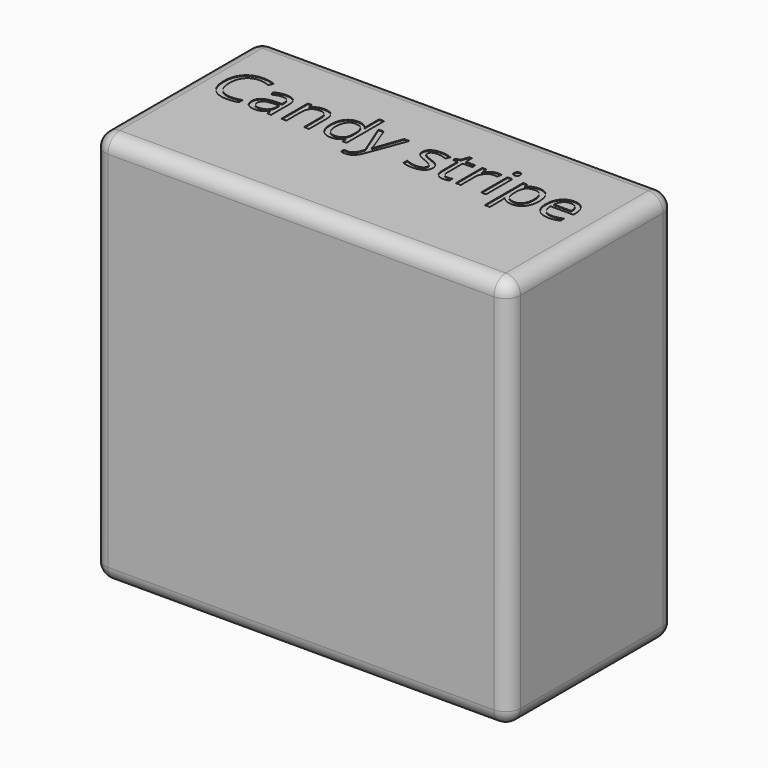
from build123d import *

# Parameters (mm, degrees)
F0_W         = 560
F0_H         = 280
F1_DEPTH     = 530
F2_R         = 20
F3_TEXT_SIZE = 83.3333333333
F4_DEPTH     = 1


# Not quite as in the source:
# - Text() gives the source's letters only with a copy of the font that has no kerning and outlines rounded to 1/6400 em; it was checked with that copy


with BuildPart() as f1:
    # F0 (on Top) → F1 (new body)
    with BuildSketch(Plane.XY):
        Rectangle(F0_W, F0_H)
    extrude(amount=F1_DEPTH)

    # F2
    f2_edges = [f1.edges().sort_by_distance(p)[0] for p in [
        (0, -140, 530),
        (280, 0, 530),
        (0, 140, 530),
        (-280, 0, 530),
        (280, 140, 265),
        (0, -140, 0),
        (280, 0, 0),
        (0, 140, 0),
        (-280, 0, 0),
        (-280, -140, 265),
        (280, -140, 265),
        (-280, 140, 265),
    ]]
    fillet(f2_edges, radius=F2_R)

    # F3 (on face) → F4 (cut)
    with BuildSketch(Plane.XY.offset(530)):
        with Locations((-250, 7.0395662842)):
            Text('Candy stripe', F3_TEXT_SIZE, font='Open Sans', text_align=(TextAlign.LEFT, TextAlign.BOTTOM))
    extrude(amount=-F4_DEPTH, mode=Mode.SUBTRACT)


solid = f1.part
